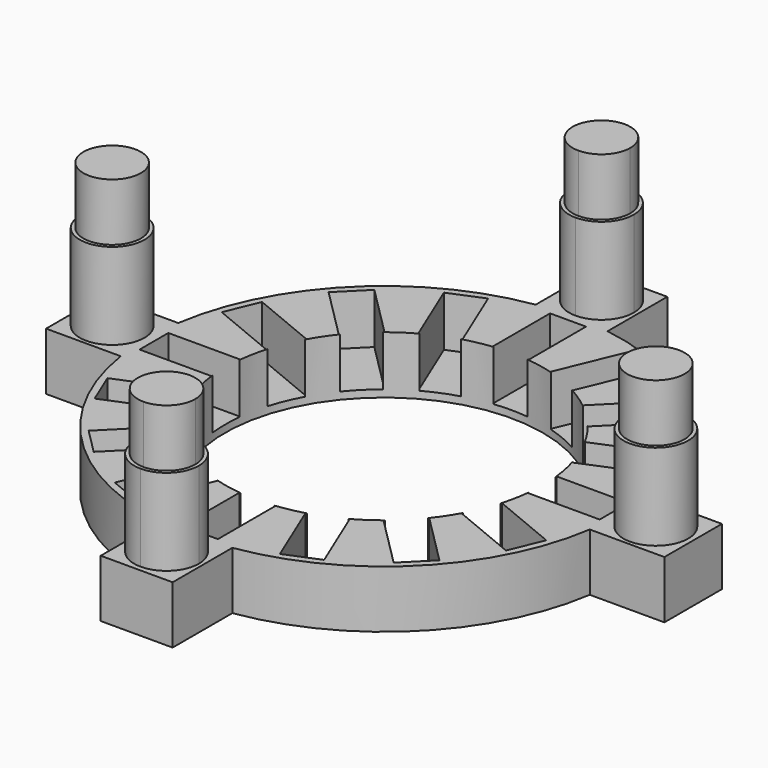
from build123d import *

# Parameters (mm, degrees)
F0_W      = 33
F0_H      = 8
F2_R      = 22.125
F3_DEPTH  = 25
F5_DEPTH  = 7
F7_DEPTH  = 8
F8_R      = 4
F9_DEPTH  = 25
F10_R     = 4.5
F10_R_2   = 4
F11_DEPTH = 20
F12_DEPTH = 28


with BuildPart() as f1:
    # F0 (on Front) → F1 (revolve)
    with BuildSketch(Plane.XZ):
        with Locations((16.5, 4)):
            Rectangle(F0_W, F0_H)
    revolve(axis=Axis((0, 0, 4), (0, 0, 1)))

    # F2 (on Top) → F3 (cut)
    with BuildSketch(Plane.XY):
        Circle(F2_R)
    extrude(amount=F3_DEPTH, mode=Mode.SUBTRACT)

    # F4 (on face) → F5 (cut)
    with BuildSketch(Plane.XY.offset(8)):
        Polygon((-2.5, 22), (0, 22), (2.5, 22), (2.5, 32), (-2.5, 32), align=None)
        Polygon((-14.555568667, 28.6074364594), (-10.7287343433, 19.3686411343), (-8.419035512, 20.3253497152), (-6.1093366808, 21.2820582962), (-9.9361710044, 30.5208536213), align=None)
        Polygon((-24.3951839509, 20.859650045), (-17.3241161391, 13.7885822331), (-15.5563491861, 15.5563491861), (-13.7885822331, 17.3241161391), (-20.859650045, 24.3951839509), align=None)
        Polygon((-30.5208536213, 9.9361710044), (-21.2820582962, 6.1093366808), (-20.3253497152, 8.419035512), (-19.3686411343, 10.7287343433), (-28.6074364594, 14.555568667), align=None)
        Polygon((-32, -2.5), (-22, -2.5), (-22, 0), (-22, 2.5), (-32, 2.5), align=None)
        Polygon((-28.6074364594, -14.555568667), (-19.3686411343, -10.7287343433), (-20.3253497152, -8.419035512), (-21.2820582962, -6.1093366808), (-30.5208536213, -9.9361710044), align=None)
        Polygon((-20.859650045, -24.3951839509), (-13.7885822331, -17.3241161391), (-15.5563491861, -15.5563491861), (-17.3241161391, -13.7885822331), (-24.3951839509, -20.859650045), align=None)
        Polygon((-9.9361710044, -30.5208536213), (-6.1093366808, -21.2820582962), (-8.419035512, -20.3253497152), (-10.7287343433, -19.3686411343), (-14.555568667, -28.6074364594), align=None)
        Polygon((2.5, -32), (2.5, -22), (0, -22), (-2.5, -22), (-2.5, -32), align=None)
        Polygon((14.555568667, -28.6074364594), (10.7287343433, -19.3686411343), (8.419035512, -20.3253497152), (6.1093366808, -21.2820582962), (9.9361710044, -30.5208536213), align=None)
        Polygon((24.3951839509, -20.859650045), (17.3241161391, -13.7885822331), (15.5563491861, -15.5563491861), (13.7885822331, -17.3241161391), (20.859650045, -24.3951839509), align=None)
        Polygon((30.5208536213, -9.9361710044), (21.2820582962, -6.1093366808), (20.3253497152, -8.419035512), (19.3686411343, -10.7287343433), (28.6074364594, -14.555568667), align=None)
        Polygon((32, 2.5), (22, 2.5), (22, 0), (22, -2.5), (32, -2.5), align=None)
        Polygon((28.6074364594, 14.555568667), (19.3686411343, 10.7287343433), (20.3253497152, 8.419035512), (21.2820582962, 6.1093366808), (30.5208536213, 9.9361710044), align=None)
        Polygon((20.859650045, 24.3951839509), (13.7885822331, 17.3241161391), (15.5563491861, 15.5563491861), (17.3241161391, 13.7885822331), (24.3951839509, 20.859650045), align=None)
        Polygon((9.9361710044, 30.5208536213), (6.1093366808, 21.2820582962), (8.419035512, 20.3253497152), (10.7287343433, 19.3686411343), (14.555568667, 28.6074364594), align=None)
    extrude(amount=-F5_DEPTH, mode=Mode.SUBTRACT)

    # F6 (on Top) → F7 (join)
    with BuildSketch(Plane.XY):
        Polygon((43, -5), (43, 0), (43, 5), (32.6190128606, 5), (32.6190128606, -5), align=None)
        Polygon((5, 32.6190128606), (5, 43), (0, 43), (-5, 43), (-5, 32.6190128606), align=None)
        Polygon((-32.6190128606, 5), (-43, 5), (-43, 0), (-43, -5), (-32.6190128606, -5), align=None)
        Polygon((-5, -32.6190128606), (-5, -43), (0, -43), (5, -43), (5, -32.6190128606), align=None)
    extrude(amount=F7_DEPTH)

    # F8 (on face) → F9 (cut)
    with BuildSketch(Plane.XY.offset(8)):
        with Locations((0, 37.8095064303)):
            Circle(F8_R)
        with Locations((37.8095064303, 0)):
            Circle(F8_R)
        with Locations((-37.8095064303, 0)):
            Circle(F8_R)
        with Locations((0, -37.8095064303)):
            Circle(F8_R)
    extrude(amount=-F9_DEPTH, mode=Mode.SUBTRACT)

    # F10 (on face) → F11 (join)
    with BuildSketch(Plane(origin=(0, 0, 0), x_dir=(1, 0, 0), z_dir=(0, 0, -1))):
        with BuildLine():
            Line((0, -41.8095064303), (0, -37.8095064303))
            Line((0, -37.8095064303), (0, -33.8095064303))
            ThreePointArc((0, -33.8095064303), (-4, -37.8095064303), (0, -41.8095064303))
        make_face()
        with BuildLine():
            Line((0, -33.8095064303), (0, -37.8095064303))
            Line((0, -37.8095064303), (0, -41.8095064303))
            ThreePointArc((0, -41.8095064303), (2.8284271247, -40.637933555), (4, -37.8095064303))
            ThreePointArc((4, -37.8095064303), (2.8284271247, -34.9810793056), (0, -33.8095064303))
        make_face()
        with BuildLine():
            ThreePointArc((42.3095064303, 0), (37.8095064303, 4.5), (33.3095064303, 0))
            ThreePointArc((33.3095064303, 0), (37.8095064303, -4.5), (42.3095064303, 0))
        make_face()
        with BuildLine():
            ThreePointArc((41.8095064303, 0), (37.8095064303, -4), (33.8095064303, 0))
            ThreePointArc((33.8095064303, 0), (37.8095064303, 4), (41.8095064303, 0))
        make_face(mode=Mode.SUBTRACT)
        with BuildLine():
            ThreePointArc((0, 41.8095064303), (-4, 37.8095064303), (0, 33.8095064303))
            Line((0, 33.8095064303), (0, 37.8095064303))
            Line((0, 37.8095064303), (0, 41.8095064303))
        make_face()
        with BuildLine():
            Line((0, 37.8095064303), (0, 33.8095064303))
            ThreePointArc((0, 33.8095064303), (2.8284271247, 34.9810793056), (4, 37.8095064303))
            ThreePointArc((4, 37.8095064303), (2.8284271247, 40.637933555), (0, 41.8095064303))
            Line((0, 41.8095064303), (0, 37.8095064303))
        make_face()
        with BuildLine():
            Line((0, -33.3095064303), (0, -33.8095064303))
            ThreePointArc((0, -33.8095064303), (2.8284271247, -34.9810793056), (4, -37.8095064303))
            ThreePointArc((4, -37.8095064303), (2.8284271247, -40.637933555), (0, -41.8095064303))
            Line((0, -41.8095064303), (0, -42.3095064303))
            ThreePointArc((0, -42.3095064303), (3.1819805153, -40.9914869456), (4.5, -37.8095064303))
            ThreePointArc((4.5, -37.8095064303), (3.1819805153, -34.627525915), (0, -33.3095064303))
        make_face()
        with BuildLine():
            ThreePointArc((0, -41.8095064303), (-4, -37.8095064303), (0, -33.8095064303))
            Line((0, -33.8095064303), (0, -33.3095064303))
            ThreePointArc((0, -33.3095064303), (-4.5, -37.8095064303), (0, -42.3095064303))
            Line((0, -42.3095064303), (0, -41.8095064303))
        make_face()
        with Locations((-37.8095064303, 0)):
            Circle(F10_R)
        with Locations((-37.8095064303, 0)):
            Circle(F10_R_2, mode=Mode.SUBTRACT)
        with BuildLine():
            ThreePointArc((0, 42.3095064303), (-4.5, 37.8095064303), (0, 33.3095064303))
            Line((0, 33.3095064303), (0, 33.8095064303))
            ThreePointArc((0, 33.8095064303), (-4, 37.8095064303), (0, 41.8095064303))
            Line((0, 41.8095064303), (0, 42.3095064303))
        make_face()
        with BuildLine():
            Line((0, 33.8095064303), (0, 33.3095064303))
            ThreePointArc((0, 33.3095064303), (3.1819805153, 34.627525915), (4.5, 37.8095064303))
            ThreePointArc((4.5, 37.8095064303), (3.1819805153, 40.9914869456), (0, 42.3095064303))
            Line((0, 42.3095064303), (0, 41.8095064303))
            ThreePointArc((0, 41.8095064303), (2.8284271247, 40.637933555), (4, 37.8095064303))
            ThreePointArc((4, 37.8095064303), (2.8284271247, 34.9810793056), (0, 33.8095064303))
        make_face()
    extrude(amount=-F11_DEPTH)

    # F10 (on face) → F12 (join)
    with BuildSketch(Plane(origin=(0, 0, 0), x_dir=(1, 0, 0), z_dir=(0, 0, -1))):
        with BuildLine():
            Line((0, -41.8095064303), (0, -37.8095064303))
            Line((0, -37.8095064303), (0, -33.8095064303))
            ThreePointArc((0, -33.8095064303), (-4, -37.8095064303), (0, -41.8095064303))
        make_face()
        with BuildLine():
            Line((0, -33.8095064303), (0, -37.8095064303))
            Line((0, -37.8095064303), (0, -41.8095064303))
            ThreePointArc((0, -41.8095064303), (2.8284271247, -40.637933555), (4, -37.8095064303))
            ThreePointArc((4, -37.8095064303), (2.8284271247, -34.9810793056), (0, -33.8095064303))
        make_face()
        with Locations((-37.8095064303, 0)):
            Circle(F10_R_2)
        with BuildLine():
            ThreePointArc((41.8095064303, 0), (37.8095064303, 4), (33.8095064303, 0))
            ThreePointArc((33.8095064303, 0), (37.8095064303, -4), (41.8095064303, 0))
        make_face()
        with BuildLine():
            ThreePointArc((0, 41.8095064303), (-4, 37.8095064303), (0, 33.8095064303))
            Line((0, 33.8095064303), (0, 37.8095064303))
            Line((0, 37.8095064303), (0, 41.8095064303))
        make_face()
        with BuildLine():
            Line((0, 37.8095064303), (0, 33.8095064303))
            ThreePointArc((0, 33.8095064303), (2.8284271247, 34.9810793056), (4, 37.8095064303))
            ThreePointArc((4, 37.8095064303), (2.8284271247, 40.637933555), (0, 41.8095064303))
            Line((0, 41.8095064303), (0, 37.8095064303))
        make_face()
    extrude(amount=-F12_DEPTH)


solid = f1.part
